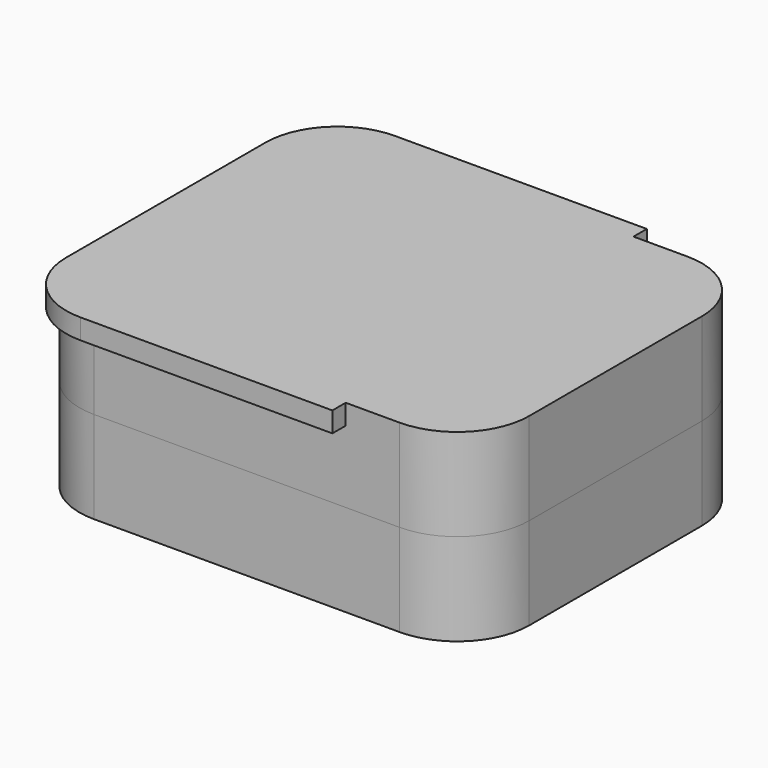
from build123d import *

# Parameters (mm, degrees)
F1_DEPTH     = 10.25
F3_DEPTH     = 2.25
F5_DEPTH     = 10.25
F6_T         = 1.9
F6_T3_DEPTH  = 31.8
F6_T5_DEPTH  = 6.05
F6_T8_ANGLE  = 90.000000001
F6_T10_ANGLE = 90.000000001
F8_DEPTH     = 2.5


# Not quite as in the source:
# - a shell that OpenCascade refuses in one call is made with other operations: the cavity is built on its own and cut out


with BuildPart() as f1:
    # F0 (on Top) → F1 (new body)
    with BuildSketch(Plane.XY):
        with BuildLine():
            Line((17, 20), (-17, 20))
            ThreePointArc((-17, 20), (-22.6568542495, 17.6568542495), (-25, 12))
            Line((-25, 12), (-25, -12))
            ThreePointArc((-25, -12), (-22.6568542495, -17.6568542495), (-17, -20))
            Line((-17, -20), (17, -20))
            ThreePointArc((17, -20), (22.6568542495, -17.6568542495), (25, -12))
            Line((25, -12), (25, 12))
            ThreePointArc((25, 12), (22.6568542495, 17.6568542495), (17, 20))
        make_face()
    extrude(amount=F1_DEPTH)

    # F2 (on face) → F3 (join)
    with BuildSketch(Plane.XY.offset(10.25)):
        with BuildLine():
            Line((11, 21.85), (-17, 21.85))
            ThreePointArc((-17, 21.85), (-22.6568542495, 19.5068542495), (-25, 13.85))
            Line((-25, 13.85), (-25, 12))
            ThreePointArc((-25, 12), (-22.6568542495, 17.6568542495), (-17, 20))
            Line((-17, 20), (11, 20))
            Line((11, 20), (11, 21.85))
        make_face()
        with BuildLine():
            Line((11, -21.85), (11, -20))
            Line((11, -20), (-17, -20))
            ThreePointArc((-17, -20), (-22.6568542495, -17.6568542495), (-25, -12))
            Line((-25, -12), (-25, -13.85))
            ThreePointArc((-25, -13.85), (-22.6568542495, -19.5068542495), (-17, -21.85))
            Line((-17, -21.85), (11, -21.85))
        make_face()
    extrude(amount=-F3_DEPTH)

    # F6: shell of thickness 1.9, made by hand


with BuildPart() as f5:
    # F4 (on face) → F5 (new body)
    with BuildSketch(Plane(origin=(0, 0, 0), x_dir=(1, 0, 0), z_dir=(0, 0, -1))):
        with BuildLine():
            Line((17, 20), (-17, 20))
            ThreePointArc((-17, 20), (-22.6568542495, 17.6568542495), (-25, 12))
            Line((-25, 12), (-25, -12))
            ThreePointArc((-25, -12), (-22.6568542495, -17.6568542495), (-17, -20))
            Line((-17, -20), (17, -20))
            ThreePointArc((17, -20), (22.6568542495, -17.6568542495), (25, -12))
            Line((25, -12), (25, 12))
            ThreePointArc((25, 12), (22.6568542495, 17.6568542495), (17, 20))
        make_face()
    extrude(amount=F5_DEPTH)


with BuildPart() as f6_core1:
    # F6_t2: copy of F1
    add(f1.part)

    # the walls: a layer under each face that stays
    f6_faces = [f6_core1.faces().sort_by_distance(p)[0] for p in [
        (0, 20, 5.125),
        (22.6568542495, 17.6568542495, 5.125),
        (25, 0, 5.125),
        (22.6568542495, -17.6568542495, 5.125),
        (0, -20, 5.125),
        (-22.6568542495, -17.6568542495, 4),
        (-25, 0, 5.125),
        (-22.6568542495, -19.5068542495, 9.125),
        (-3, -21.85, 9.125),
        (-22.6568542495, 19.5068542495, 9.125),
        (-3, 21.85, 9.125),
        (-19, -20.2083333333, 8),
        (11, -20.925, 9.125),
        (0, 0, 10.25),
        (11, 20.925, 9.125),
        (-19, 20.2083333333, 8),
        (-22.6568542495, 17.6568542495, 4),
    ]]
    thicken(f6_faces, amount=-F6_T, mode=Mode.SUBTRACT)

    # F6_s4 → F6_t3 (cut)
    with BuildSketch(Plane.YZ.offset(-18.9)):
        Polygon((20.019, 7.981), (18.1, 8), (18.1, 9.9), (20, 9.9), align=None)
        Polygon((-20.019, 7.981), (-18.1, 8), (-18.1, 9.9), (-20, 9.9), align=None)
    extrude(amount=F6_T3_DEPTH, mode=Mode.SUBTRACT)

    # F6_s6 → F6_t5 (cut)
    with BuildSketch(Plane.XY.offset(6.1)):
        Polygon((11.019, 20.019), (11, 18.1), (9.1, 18.1), (9.1, 20), align=None)
        Polygon((11.019, -20.019), (11, -18.1), (9.1, -18.1), (9.1, -20), align=None)
    extrude(amount=F6_T5_DEPTH, mode=Mode.SUBTRACT)

    # F6_s7 → F6_t8 (revolve, cut)
    with BuildSketch(Plane.YZ.offset(-17)):
        Polygon((-20.019, 7.981), (-18.1, 8), (-18.1, 9.9), (-20, 9.9), align=None)
    revolve(axis=Axis((-17, -12, 8), (0, 0, -1)), revolution_arc=F6_T8_ANGLE, mode=Mode.SUBTRACT)

    # F6_s9 → F6_t10 (revolve, cut)
    with BuildSketch(Plane.XZ.offset(-12)):
        Polygon((-25.019, 7.981), (-25, 9.9), (-23.1, 9.9), (-23.1, 8), align=None)
    revolve(axis=Axis((-17, 12, 8), (0, 0, -1)), revolution_arc=F6_T10_ANGLE, mode=Mode.SUBTRACT)


with BuildPart() as f1_1:
    add(f1.part)

    # what is left inside the walls is the cavity
    f6_cavity = [f6_core1.part.solids().sort_by_distance(p)[0] for p in [
        (0, -6.033333, 8.331),
    ]]
    add(f6_cavity, mode=Mode.SUBTRACT)

    # F7 (on face) → F8 (cut)
    with BuildSketch(Plane(origin=(0, 0, 0), x_dir=(1, 0, 0), z_dir=(0, 0, -1))):
        with BuildLine():
            ThreePointArc((-17, 19.1), (-22.0204581464, 17.0204581464), (-24.1, 12))
            Line((-24.1, 12), (-24.1, -12))
            ThreePointArc((-24.1, -12), (-22.0204581464, -17.0204581464), (-17, -19.1))
            Line((-17, -19.1), (17, -19.1))
            ThreePointArc((17, -19.1), (22.0204581464, -17.0204581464), (24.1, -12))
            Line((24.1, -12), (24.1, 12))
            ThreePointArc((24.1, 12), (22.0204581464, 17.0204581464), (17, 19.1))
            Line((17, 19.1), (-17, 19.1))
        make_face()
        with BuildLine():
            Line((-23.1, -12), (-23.1, 12))
            ThreePointArc((-23.1, 12), (-21.3133513652, 16.3133513652), (-17, 18.1))
            Line((-17, 18.1), (17, 18.1))
            ThreePointArc((17, 18.1), (21.3133513652, 16.3133513652), (23.1, 12))
            Line((23.1, 12), (23.1, -12))
            ThreePointArc((23.1, -12), (21.3133513652, -16.3133513652), (17, -18.1))
            Line((17, -18.1), (-17, -18.1))
            ThreePointArc((-17, -18.1), (-21.3133513652, -16.3133513652), (-23.1, -12))
        make_face(mode=Mode.SUBTRACT)
    extrude(amount=-F8_DEPTH, mode=Mode.SUBTRACT)


solid = Compound([f5.part, f1_1.part])
